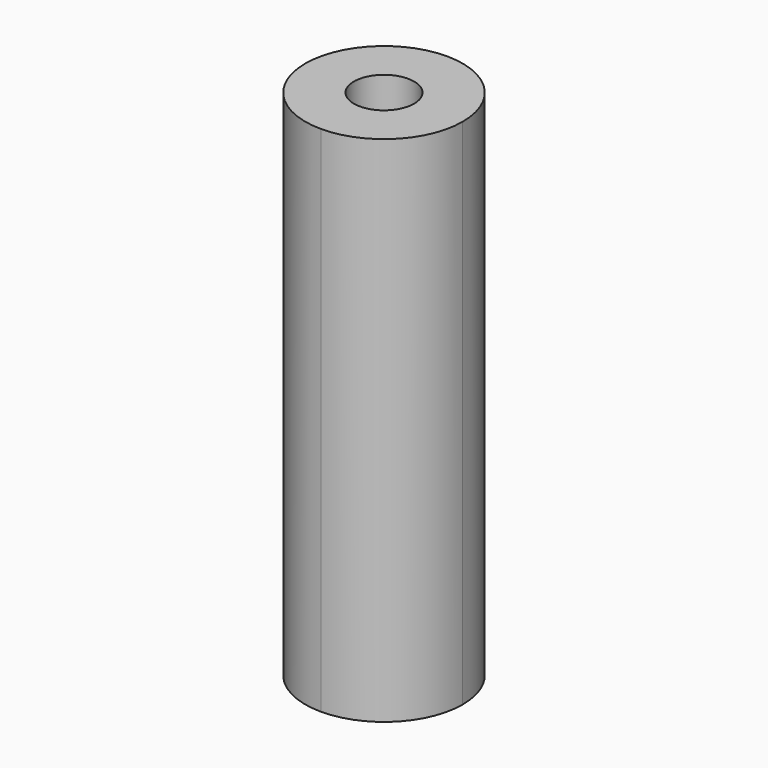
from build123d import *

# Parameters (mm, degrees)
F0_W        = 11.2655872395
F0_H        = 11.2655872395
F0_R        = 2.15265
F1_DEPTH    = 22.4125
F2_W        = 11.2655872395
F2_H        = 11.2655872395
F3_DEPTH    = 1.5875
F4_W        = 11.2655872395
F4_H        = 11.2655872395
F4_R        = 2.15265
F5_DEPTH    = 12.7
F6_R        = 1.35255
F7_DEPTH    = 4.9581264334
F8_T1_DEPTH = 64.8639645


# Not quite as in the source:
# - a fillet or chamfer that OpenCascade refuses, or shapes differently, is made with other operations: its cross-section is extruded or revolved along the edge and cut away or added


with BuildPart() as f1:
    # F0 (on Top) → F1 (new body)
    with BuildSketch(Plane.XY):
        Rectangle(F0_W, F0_H)
        Circle(F0_R, mode=Mode.SUBTRACT)
    extrude(amount=F1_DEPTH)

    # F2 (on face) → F3 (join)
    with BuildSketch(Plane.XY.offset(22.4125)):
        Rectangle(F2_W, F2_H)
    extrude(amount=F3_DEPTH)

    # F4 (on face) → F5 (join)
    with BuildSketch(Plane.XY.offset(24)):
        Rectangle(F4_W, F4_H)
        Circle(F4_R, mode=Mode.SUBTRACT)
    extrude(amount=F5_DEPTH)

    # F6 (on face) → F7 (cut, up to face)
    with BuildSketch(Plane(origin=(-5.6327936197, 0, 0), x_dir=(0, -1, 0), z_dir=(-1, 0, 0))):
        with Locations((0, 11.20625)):
            Circle(F6_R)
        with Locations((0, 30.35)):
            Circle(F6_R)
    extrude(amount=-F7_DEPTH, mode=Mode.SUBTRACT)

    # F8: fillet of radius 5.6327929 on 4 edges, made by hand

    # F8_s2 → F8_t1 (cut)
    with BuildSketch(Plane.XY.offset(-14.08198225)):
        with BuildLine():
            ThreePointArc((-5.6327936197, 7.197e-07), (-3.9829867763, 3.9829867763), (-7.197e-07, 5.6327936197))
            Line((-7.197e-07, 5.6327936197), (-5.6327936197, 5.6327936197))
            Line((-5.6327936197, 5.6327936197), (-5.6327936197, 7.197e-07))
        make_face()
        with BuildLine():
            ThreePointArc((5.6327936197, 7.197e-07), (3.9829867763, 3.9829867763), (7.197e-07, 5.6327936197))
            Line((7.197e-07, 5.6327936197), (5.6327936197, 5.6327936197))
            Line((5.6327936197, 5.6327936197), (5.6327936197, 7.197e-07))
        make_face()
        with BuildLine():
            ThreePointArc((-7.197e-07, -5.6327936197), (-3.9829867763, -3.9829867763), (-5.6327936197, -7.197e-07))
            Line((-5.6327936197, -7.197e-07), (-5.6327936197, -5.6327936197))
            Line((-5.6327936197, -5.6327936197), (-7.197e-07, -5.6327936197))
        make_face()
        with BuildLine():
            ThreePointArc((7.197e-07, -5.6327936197), (3.9829867763, -3.9829867763), (5.6327936197, -7.197e-07))
            Line((5.6327936197, -7.197e-07), (5.6327936197, -5.6327936197))
            Line((5.6327936197, -5.6327936197), (7.197e-07, -5.6327936197))
        make_face()
    extrude(amount=F8_T1_DEPTH, mode=Mode.SUBTRACT)


solid = f1.part
